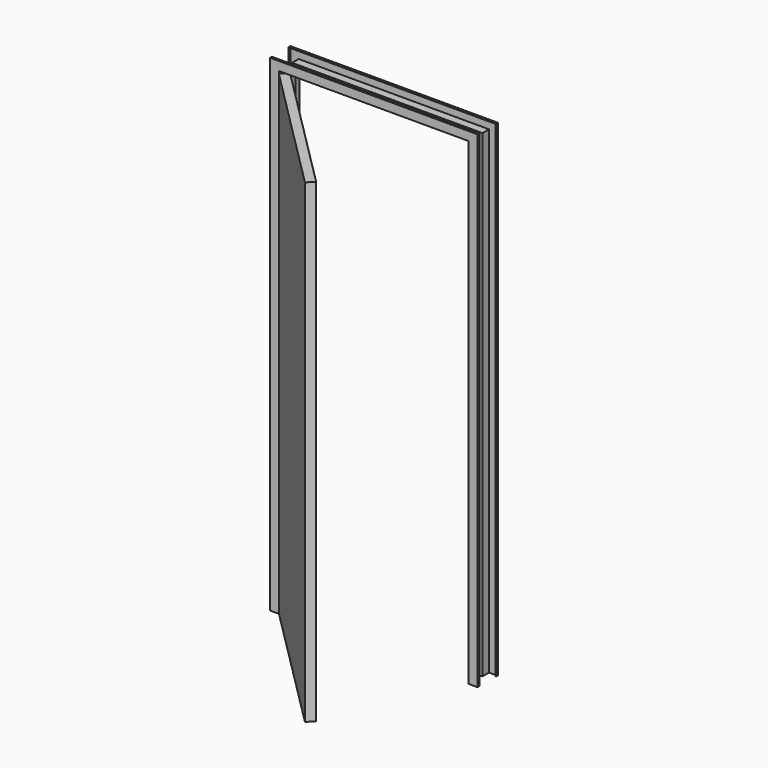
from build123d import *

# Parameters (mm, degrees)
F5_DEPTH = 1370.0125


# Not quite as in the source:
# - a variable given as a bare number and used for a length is read in inches; the dataset says mm whatever the document's units were


with BuildPart() as f3:
    # F3: sweep along a path in F1
    with BuildLine(Plane.XZ) as f3_path:
        Line((-533.4, -1371.6), (-533.4, 1371.6))
        Line((-533.4, 1371.6), (533.4, 1371.6))
        Line((533.4, 1371.6), (533.4, -1371.6))
    # F2 (on Top) → F3 (sweep)
    with BuildSketch(Plane.XY):
        Polygon((-549.275, 23.368), (-533.4, 23.368), (-533.4, -23.368), (-549.275, -23.368), (-549.275, -70.993), (-596.011, -70.993), (-596.011, -60.325), (-598.043, -60.325), (-598.043, -73.025), (-547.243, -73.025), (-547.243, -25.4), (-531.368, -25.4), (-531.368, 25.4), (-547.243, 25.4), (-547.243, 73.025), (-598.043, 73.025), (-598.043, 60.325), (-596.011, 60.325), (-596.011, 70.993), (-549.275, 70.993), align=None)
    sweep(path=f3_path.line, transition=Transition.RIGHT)

    # F4 (on Top) → F5 (join, symmetric)
    with BuildSketch(Plane.XY):
        Polygon((240.1792460268, -789.4134896855), (-514.1622681431, -35.0719755157), (-550.0832926273, -70.993), (204.2582215425, -825.3345141698), align=None)
    extrude(amount=F5_DEPTH, both=True)


solid = f3.part
